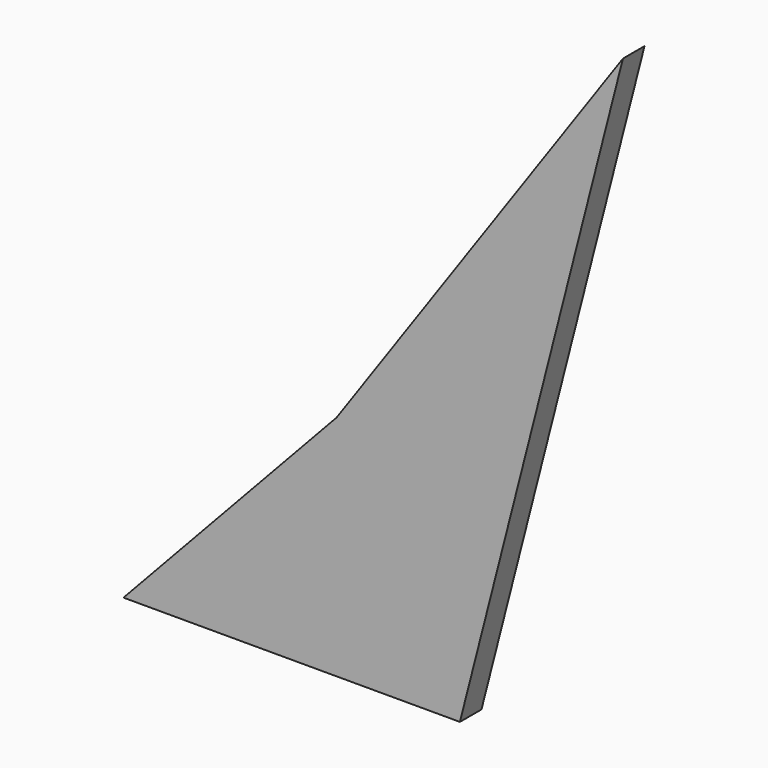
from build123d import *

# Parameters (mm, degrees)
F1_DEPTH = 3.81


# Not quite as in the source:
# - a feature names something its author has since deleted; it is built from what else it names


with BuildPart() as f1:
    # F0 (on Front) → F1 (new body)
    with BuildSketch(Plane.XZ):
        Polygon((22.4553077279, 121.7113970666), (-18.0439893156, 63.8412535191), (-48.184117534, 31.6155430744), (-0.604117534, 31.6155430744), align=None)
    extrude(amount=F1_DEPTH)


solid = f1.part
